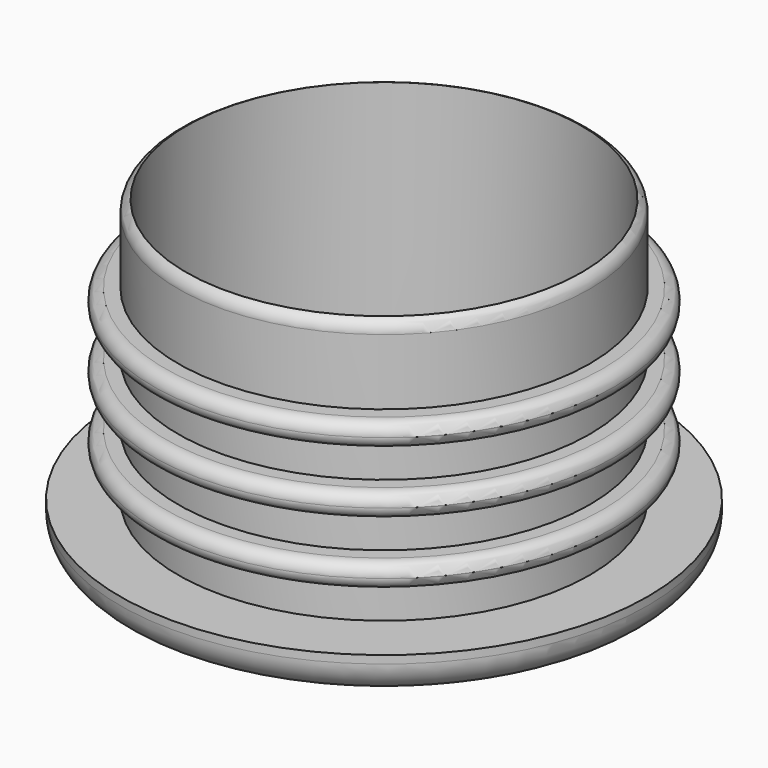
from build123d import *

# Parameters (mm, degrees)
F0_R      = 19.812
F0_R_2    = 19.05
F1_DEPTH  = 29.21
F0_R_3    = 25.4
F2_DEPTH  = 3.81
F6_R      = 22.225
F6_R_2    = 19.05
F9_DEPTH  = 1.143
F7_R      = 22.225
F7_R_2    = 19.05
F10_DEPTH = 1.143
F8_R      = 22.225
F8_R_2    = 19.05
F11_DEPTH = 1.143
F12_R     = 3.048
F14_R     = 1.14299
F15_R     = 1.14299
F16_R     = 1.14299


# Not quite as in the source:
# - a fillet or chamfer that OpenCascade refuses, or shapes differently, is made with other operations: its cross-section is extruded or revolved along the edge and cut away or added
# - a fillet or chamfer is up to 0.001 mm smaller than in the source, because OpenCascade refuses the exact size


with BuildPart() as f1:
    # F0 (on Top) → F1 (new body)
    with BuildSketch(Plane.XY):
        Circle(F0_R)
        Circle(F0_R_2, mode=Mode.SUBTRACT)
    extrude(amount=F1_DEPTH)

    # F0 (on Top) → F2 (join)
    with BuildSketch(Plane.XY):
        Circle(F0_R_3)
        Circle(F0_R, mode=Mode.SUBTRACT)
        Circle(F0_R)
        Circle(F0_R_2, mode=Mode.SUBTRACT)
        Circle(F0_R_2)
    extrude(amount=F2_DEPTH)

    # F6 (on offset) → F9 (join, symmetric)
    with BuildSketch(Plane.XY.offset(8.636)):
        Circle(F6_R)
        Circle(F6_R_2, mode=Mode.SUBTRACT)
    extrude(amount=F9_DEPTH, both=True)

    # F7 (on offset) → F10 (join, symmetric)
    with BuildSketch(Plane.XY.offset(14.605)):
        Circle(F7_R)
        Circle(F7_R_2, mode=Mode.SUBTRACT)
    extrude(amount=F10_DEPTH, both=True)

    # F8 (on offset) → F11 (join, symmetric)
    with BuildSketch(Plane.XY.offset(20.574)):
        Circle(F8_R)
        Circle(F8_R_2, mode=Mode.SUBTRACT)
    extrude(amount=F11_DEPTH, both=True)

    # F12
    f12_edges = [f1.edges().sort_by_distance(p)[0] for p in [
        (-25.4, 0, 0),
    ]]
    fillet(f12_edges, radius=F12_R)

    # F13: fillet of radius 1.27 on 1 edges, made by hand

    # F13_s1 → F13_t2 (revolve, cut)
    with BuildSketch(Plane.XZ):
        with BuildLine():
            ThreePointArc((19.812, 28.0460257735), (19.6045582337, 28.7416334215), (19.05, 29.21))
            Line((19.05, 29.21), (19.812, 29.21))
            Line((19.812, 29.21), (19.812, 28.0460257735))
        make_face()
    revolve(axis=Axis((0, 0, 29.21), (0, 0, 1)), mode=Mode.SUBTRACT)

    # F14 (radius 1.143 in the source; OpenCascade refuses exactly that, so slightly less here)
    f14_edges = [f1.edges().sort_by_distance(p)[0] for p in [
        (-22.225, 0, 7.493),
        (-22.225, 0, 9.779),
    ]]
    fillet(f14_edges, radius=F14_R)

    # F15 (radius 1.143 in the source; OpenCascade refuses exactly that, so slightly less here)
    f15_edges = [f1.edges().sort_by_distance(p)[0] for p in [
        (-22.225, 0, 13.462),
        (-22.225, 0, 15.748),
    ]]
    fillet(f15_edges, radius=F15_R)

    # F16 (radius 1.143 in the source; OpenCascade refuses exactly that, so slightly less here)
    f16_edges = [f1.edges().sort_by_distance(p)[0] for p in [
        (-22.225, 0, 19.431),
        (-22.225, 0, 21.717),
    ]]
    fillet(f16_edges, radius=F16_R)


solid = f1.part
